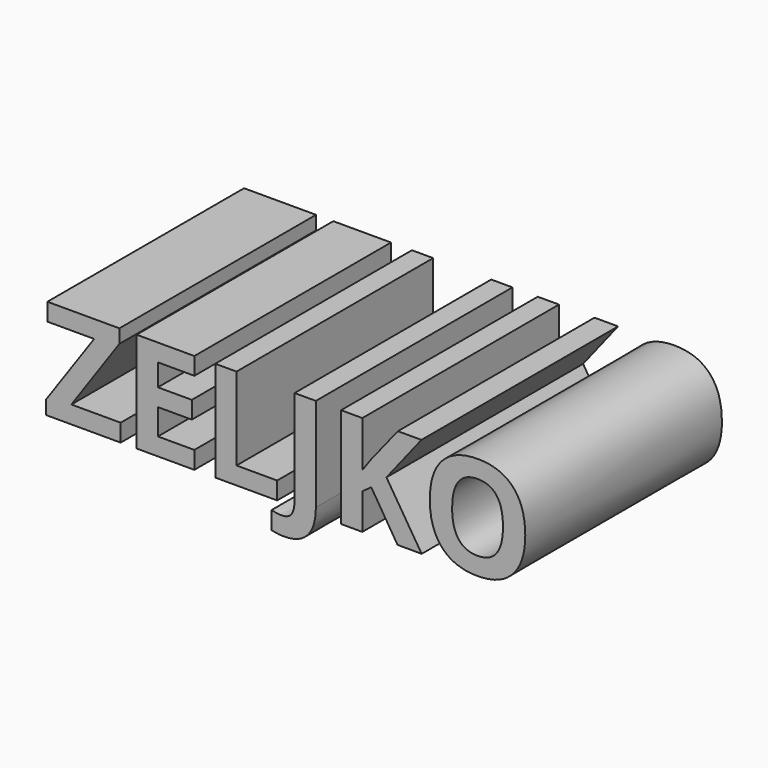
from build123d import *

# Parameters (mm, degrees)
F0_TEXT_SIZE = 28.5561306443
F1_DEPTH     = 50


# Not quite as in the source:
# - Text() gives the source's letters only with a copy of the font that has no kerning and outlines rounded to 1/6400 em; it was checked with that copy


with BuildPart() as f1:
    # F0 (on Front) → F1 (new body)
    with BuildSketch(Plane.XZ):
        with Locations((-57.9555645838, 13.6327760071)):
            Text('ZELJKO', F0_TEXT_SIZE, font='Open Sans', font_style=FontStyle.BOLD, text_align=(TextAlign.LEFT, TextAlign.BOTTOM))
    extrude(amount=F1_DEPTH)


solid = f1.part
